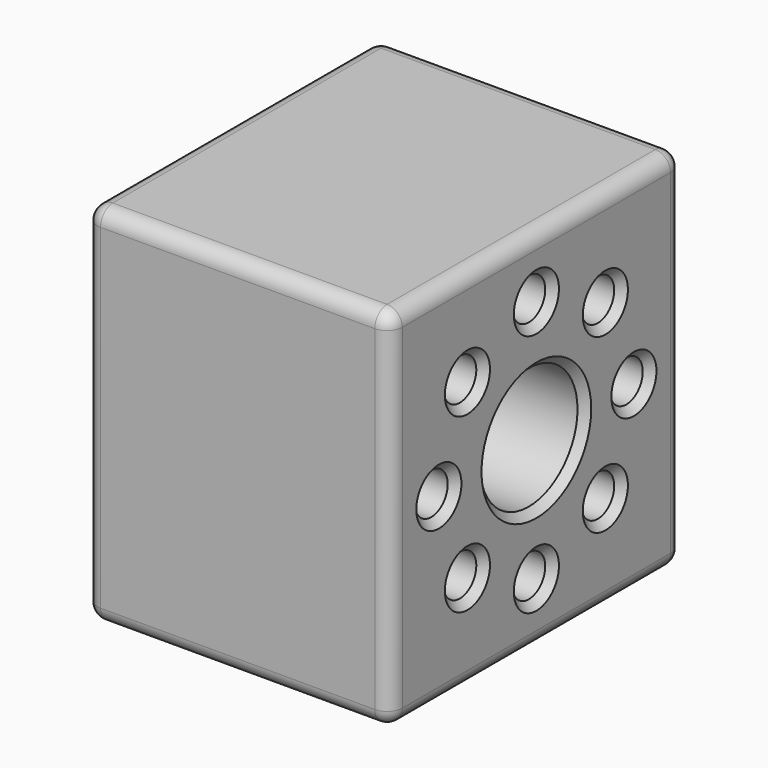
from build123d import *

# Parameters (mm, degrees)
F0_W     = 20
F0_H     = 24
F1_DEPTH = 24
F2_R     = 4
F3_DEPTH = 20.001
F5_D     = 2.7051
F5_DEPTH = 6
F5_TIP   = 0.8126940303
F7_D     = 2.7051
F7_DEPTH = 6
F7_TIP   = 0.8126940303
F8_R     = 1
F9_SIZE  = 0.5


with BuildPart() as f1:
    # F0 (on Top) → F1 (new body)
    with BuildSketch(Plane.XY):
        Rectangle(F0_W, F0_H)
    extrude(amount=F1_DEPTH)

    # F2 (on face) → F3 (cut, through all)
    with BuildSketch(Plane.YZ.offset(10)):
        with Locations((0, 12)):
            Circle(F2_R)
    extrude(amount=-F3_DEPTH, mode=Mode.SUBTRACT)

    # F5
    with Locations(Plane.YZ.offset(10)):
        with Locations((0, 20), (5.6568542495, 17.6568542495), (8, 12), (5.6568542495, 6.3431457505), (0, 4), (-5.6568542495, 6.3431457505), (-8, 12), (-5.6568542495, 17.6568542495)):
            Hole(F5_D / 2, depth=F5_DEPTH)
            with Locations((0, 0, -(F5_DEPTH + F5_TIP / 2))):  # 118° drill point
                Cone(0, F5_D / 2, F5_TIP, mode=Mode.SUBTRACT)

    # F7
    with Locations(Plane(origin=(-10, 0, 0), x_dir=(0, -1, 0), z_dir=(-1, 0, 0))):
        with Locations((0, 20), (5.6568542495, 17.6568542495), (8, 12), (5.6568542495, 6.3431457505), (0, 4), (-5.6568542495, 6.3431457505), (-8, 12), (-5.6568542495, 17.6568542495)):
            Hole(F7_D / 2, depth=F7_DEPTH)
            with Locations((0, 0, -(F7_DEPTH + F7_TIP / 2))):  # 118° drill point
                Cone(0, F7_D / 2, F7_TIP, mode=Mode.SUBTRACT)

    # F8
    f8_edges = [f1.edges().sort_by_distance(p)[0] for p in [
        (0, -12, 24),
        (10, 0, 24),
        (0, 12, 24),
        (-10, 0, 24),
        (-10, -12, 12),
        (10, -12, 12),
        (0, -12, 0),
        (10, 12, 12),
        (-10, 12, 12),
        (0, 12, 0),
        (10, 0, 0),
        (-10, 0, 0),
    ]]
    fillet(f8_edges, radius=F8_R)

    # F9
    f9_edges = [f1.edges().sort_by_distance(p)[0] for p in [
        (10, -4, 12),
        (-10, -4, 12),
        (-10, 7.009404, 17.656854),
        (-10, 1.35255, 20),
        (-10, -4.304304, 17.656854),
        (-10, 9.35255, 12),
        (-10, 7.009404, 6.343146),
        (-10, -6.64745, 12),
        (-10, 1.35255, 4),
        (-10, -4.304304, 6.343146),
        (10, -7.009404, 17.656854),
        (10, -1.35255, 20),
        (10, 4.304304, 17.656854),
        (10, -9.35255, 12),
        (10, -7.009404, 6.343146),
        (10, 6.64745, 12),
        (10, -1.35255, 4),
        (10, 4.304304, 6.343146),
    ]]
    chamfer(f9_edges, length=F9_SIZE)


solid = f1.part
